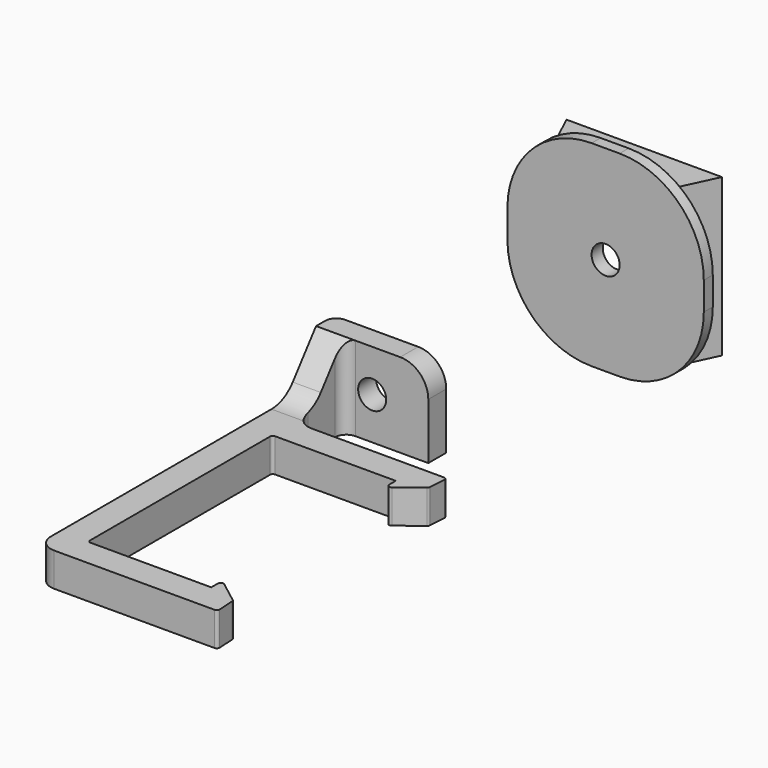
from build123d import *

# Parameters (mm, degrees)
F1_DEPTH     = 6
F3_DEPTH     = 15
F5_DEPTH     = 5.0000008951
F6_R         = 5
F10_DEPTH    = 5
F11_W        = 35
F11_H        = 35
F12_DEPTH    = 2
F15_W        = 27.7
F15_H        = 28
F13_W        = 21.5
F13_H        = 28
F17_T        = 2.5
F17_T3_DEPTH = 26.5
F17_T5_DEPTH = 33
F19_R        = 2.5
F20_DEPTH    = 54.5
F21_R        = 15
F22_R        = 3
F23_R        = 0.5
F24_R        = 2
F25_R        = 6


# Not quite as in the source:
# - ends of sketch curves that miss each other by under 0.0002 mm in the source are joined
# - a shell that OpenCascade refuses in one call is made with other operations: the cavity is built on its own and cut out


with BuildPart() as f1:
    # F0 (on Top) → F1 (new body)
    with BuildSketch(Plane.XY):
        Polygon((11.0000005256, -18.05), (11.0000005256, -20.55), (-11.0000005256, -20.55), (-10.9999994744, 20.55), (11.0000005256, 20.55), (11.0000005256, 18.05), (15.8927322497, 21.8000001848), (16.1137396651, 25.5500003695), (11.4420153564, 25.5500003695), (-15.9999997161, 25.5500003695), (-16.000001023, -25.5500003695), (11.4420153564, -25.5500003695), (16.1137396651, -25.5500003695), (15.8927322497, -21.8000001848), align=None)
    extrude(amount=F1_DEPTH)

    # F2 (on face) → F3 (join)
    with BuildSketch(Plane(origin=(0, 0, 0), x_dir=(1, 0, 0), z_dir=(0, 0, -1))):
        Polygon((-10.9999994744, -25.5500003695), (-15.9999997161, -25.5500003695), (-15.9999997161, -40.5500003695), (-10.9999994744, -40.5500003695), (4.0000002839, -40.5500003695), (4.0000002839, -36.5500003695), (-10.9999994744, -36.5500003695), align=None)
    extrude(amount=-F3_DEPTH)

    # F4 (on face) → F5 (cut, through all)
    with BuildSketch(Plane.YZ.offset(-10.9999994744)):
        Polygon((25.5500003695, 15), (25.5500003695, 6), (29.5500003695, 6), (36.5500003695, 15), align=None)
    extrude(amount=-F5_DEPTH, mode=Mode.SUBTRACT)

    # F6
    f6_edges = [f1.edges().sort_by_distance(p)[0] for p in [
        (4, 38.55, 15),
    ]]
    fillet(f6_edges, radius=F6_R)


with BuildPart() as f10:
    # F9 (on offset) → F10 (new body)
    with BuildSketch(Plane(origin=(0, 65.5500003695, 0), x_dir=(-1, 0, 0), z_dir=(0, 1, 0))):
        with BuildLine():
            Line((15.9999997161, 0), (15.9999997161, 15))
            Line((15.9999997161, 15), (0.9999997161, 15))
            ThreePointArc((0.9999997161, 15), (-2.5355341898, 13.5355339059), (-4.0000002839, 10))
            Line((-4.0000002839, 10), (-4.0000002839, 0))
            Line((-4.0000002839, 0), (15.9999997161, 0))
        make_face()
    extrude(amount=F10_DEPTH)


with BuildPart() as f12:
    # F11 (on offset) → F12 (new body)
    with BuildSketch(Plane(origin=(0, 88.5500003695, 0), x_dir=(-1, 0, 0), z_dir=(0, 1, 0))):
        with Locations((5.9999997161, 7.5)):
            Rectangle(F11_W, F11_H)
    extrude(amount=F12_DEPTH)

    # F15 (on offset) → F16 section 0
    with BuildSketch(Plane(origin=(0, 97.1500003695, 0), x_dir=(-1, 0, 0), z_dir=(0, 1, 0))):
        with Locations((5.9999997161, 7.5)):
            Rectangle(F15_W, F15_H)
    # F13 (on face) → F16 section 1
    with BuildSketch(Plane(origin=(0, 90.5500003695, 0), x_dir=(-1, 0, 0), z_dir=(0, 1, 0))):
        with Locations((5.9999997161, 7.5)):
            Rectangle(F13_W, F13_H)
    loft()

    # F17: shell of thickness 2.5, made by hand


with BuildPart() as f17_core1:
    # F17_t2: copy of F12
    add(f12.part)

    # the walls: a layer under each face that stays
    f17_faces = [f17_core1.faces().sort_by_distance(p)[0] for p in [
        (-5.9999997161, 89.5500003695, -10),
        (11.5000002839, 89.5500003695, 7.5),
        (-23.4999997161, 89.5500003695, 7.5),
        (-5.9999997161, 88.5500003695, 7.5),
        (5.6666669506, 90.5500003695, -4.1666666667),
        (-5.9999997161, 89.5500003695, 25),
        (-5.9999997161, 93.8500003695, -6.5),
        (-18.2999997161, 93.8500003695, 7.5),
        (-5.9999997161, 93.8500003695, 21.5),
        (6.3000002839, 93.8500003695, 7.5),
    ]]
    thicken(f17_faces, amount=-F17_T, mode=Mode.SUBTRACT)

    # F17_s4 → F17_t3 (cut)
    with BuildSketch(Plane.YZ.offset(-19.2499997161)):
        Polygon((90.5750003695, -6.525), (88.0500003695, -6.5), (88.0500003695, -4), (90.5500003695, -4), align=None)
        Polygon((90.5750003695, 21.525), (88.0500003695, 21.5), (88.0500003695, 19), (90.5500003695, 19), align=None)
    extrude(amount=F17_T3_DEPTH, mode=Mode.SUBTRACT)

    # F17_s6 → F17_t5 (cut)
    with BuildSketch(Plane.XY.offset(-9)):
        Polygon((-16.7726279476, 90.5643719578), (-16.7499997161, 88.0500003695), (-12.8137208564, 88.0500003695), (-14.4871765615, 91.6128415482), align=None)
        Polygon((4.7726285154, 90.5643719578), (4.7500002839, 88.0500003695), (0.8137214242, 88.0500003695), (2.4871771293, 91.6128415482), align=None)
    extrude(amount=F17_T5_DEPTH, mode=Mode.SUBTRACT)


with BuildPart() as f12_1:
    add(f12.part)

    # what is left inside the walls is the cavity
    f17_cavity = [f17_core1.part.solids().sort_by_distance(p)[0] for p in [
        (-2.215544, 97.125, 11.243908),
    ]]
    add(f17_cavity, mode=Mode.SUBTRACT)


with BuildPart() as f20_tool:
    # F19 (on face) → F20 (new body, through all)
    with BuildSketch(Plane(origin=(0, 91.0500003695, 0), x_dir=(-1, 0, 0), z_dir=(0, 1, 0))):
        with Locations((5.9999997161, 7.5)):
            Circle(F19_R)
    extrude(amount=-F20_DEPTH)


with BuildPart() as f1_1:
    add(f1.part)

    # F20: cut by f20_tool
    add(f20_tool.part, mode=Mode.SUBTRACT)

    # F22
    f22_edges = [f1_1.edges().sort_by_distance(p)[0] for p in [
        (-16.000001, -25.55, 3),
        (-10.999999, 25.55, 3),
    ]]
    fillet(f22_edges, radius=F22_R)

    # F23
    f23_edges = [f1_1.edges().sort_by_distance(p)[0] for p in [
        (11.000001, -18.05, 3),
        (11.000001, 18.05, 3),
        (-10.999999, 20.55, 3),
        (-11.000001, -20.55, 3),
        (16.11374, 25.55, 3),
        (15.892732, 21.8, 3),
        (15.892732, -21.8, 3),
        (16.11374, -25.55, 3),
    ]]
    fillet(f23_edges, radius=F23_R)

    # F24
    f24_edges = [f1_1.edges().sort_by_distance(p)[0] for p in [
        (-16, 40.55, 7.5),
        (-10.999999, 36.55, 7.5),
    ]]
    fillet(f24_edges, radius=F24_R)

    # F25
    f25_edges = [f1_1.edges().sort_by_distance(p)[0] for p in [
        (-13.5, 29.55, 6),
    ]]
    fillet(f25_edges, radius=F25_R)


with BuildPart() as f12_2:
    add(f12_1.part)

    # F20: cut by f20_tool
    add(f20_tool.part, mode=Mode.SUBTRACT)

    # F21
    f21_edges = [f12_2.edges().sort_by_distance(p)[0] for p in [
        (11.5, 89.55, 25),
        (-23.5, 89.55, 25),
        (-23.5, 89.55, -10),
        (11.5, 89.55, -10),
    ]]
    fillet(f21_edges, radius=F21_R)


solid = Compound([f1_1.part, f12_2.part])
